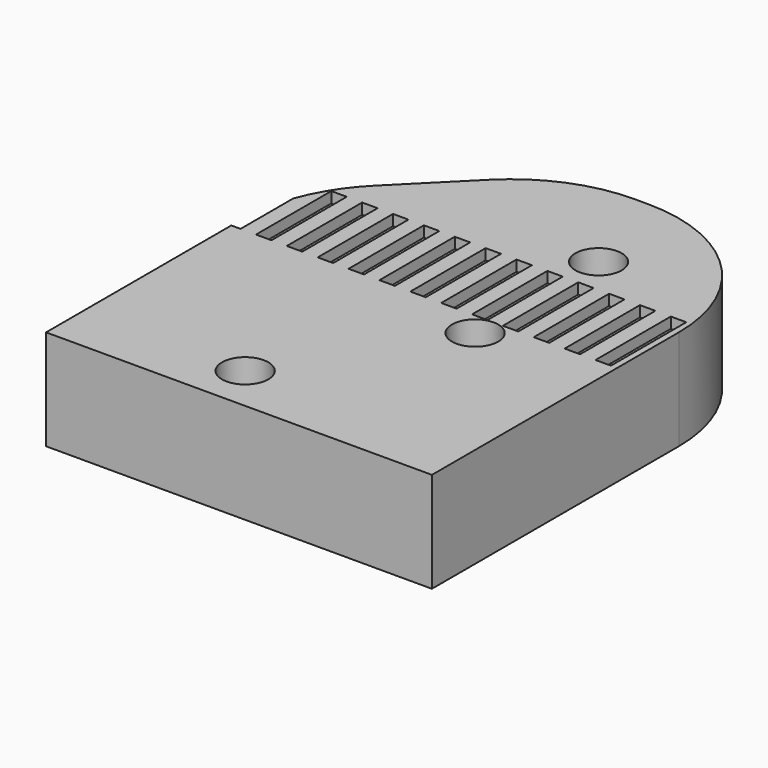
from build123d import *

# Parameters (mm, degrees)
F0_W        = 25
F0_H        = 30
F1_DEPTH    = 6.5
F2_R        = 1.5
F3_DEPTH    = 6.501
F4_W        = 1
F4_H        = 6.1
F4_W_2      = 0.4
F4_W_3      = 0.6
F5_DEPTH    = 0.7
F6_T1_DEPTH = 57.9336597593
F7_R        = 10


# Not quite as in the source:
# - a fillet or chamfer that OpenCascade refuses, or shapes differently, is made with other operations: its cross-section is extruded or revolved along the edge and cut away or added


with BuildPart() as f1:
    # F0 (on Top) → F1 (new body)
    with BuildSketch(Plane.XY):
        Rectangle(F0_W, F0_H)
    extrude(amount=F1_DEPTH)

    # F2 (on face) → F3 (cut, through all)
    with BuildSketch(Plane.XY.offset(6.5)):
        with Locations((-2, -12)):
            Circle(F2_R)
        with Locations((4.5, -1.5)):
            Circle(F2_R)
        with Locations((4.5, 8.5)):
            Circle(F2_R)
    extrude(amount=-F3_DEPTH, mode=Mode.SUBTRACT)

    # F4 (on face) → F5 (cut)
    with BuildSketch(Plane.XY.offset(6.5)):
        with Locations((11.6, 3.051)):
            Rectangle(F4_W, F4_H)
        with Locations((9.6, 3.051)):
            Rectangle(F4_W, F4_H)
        with Locations((7.6, 3.051)):
            Rectangle(F4_W, F4_H)
        with Locations((5.6, 3.051)):
            Rectangle(F4_W, F4_H)
        with Locations((3.6, 3.051)):
            Rectangle(F4_W, F4_H)
        with Locations((1.6, 3.051)):
            Rectangle(F4_W, F4_H)
        with Locations((-0.4, 3.051)):
            Rectangle(F4_W, F4_H)
        with Locations((-2.4, 3.051)):
            Rectangle(F4_W, F4_H)
        with Locations((-4.4, 3.051)):
            Rectangle(F4_W, F4_H)
        with Locations((-6.4, 3.051)):
            Rectangle(F4_W, F4_H)
        with Locations((-8.4, 3.051)):
            Rectangle(F4_W, F4_H)
        with Locations((-10.4, 3.051)):
            Rectangle(F4_W, F4_H)
        with Locations((-12.7, 3.051)):
            Rectangle(F4_W_2, F4_H)
        with Locations((-12.2, 3.051)):
            Rectangle(F4_W_3, F4_H)
    extrude(amount=-F5_DEPTH, mode=Mode.SUBTRACT)

    # F6: chamfer of 10 on 1 edges, made by hand

    # F6_s2 → F6_t1 (cut)
    with BuildSketch(Plane.XY.offset(-25.7168298797)):
        Polygon((-12.5, 5), (-2.5, 15), (-12.5, 15), align=None)
    extrude(amount=F6_T1_DEPTH, mode=Mode.SUBTRACT)

    # F7
    f7_edges = [f1.edges().sort_by_distance(p)[0] for p in [
        (-2.5, 15, 3.25),
        (-12.5, 5, 2.9),
        (12.5, 15, 3.25),
    ]]
    fillet(f7_edges, radius=F7_R)


solid = f1.part
